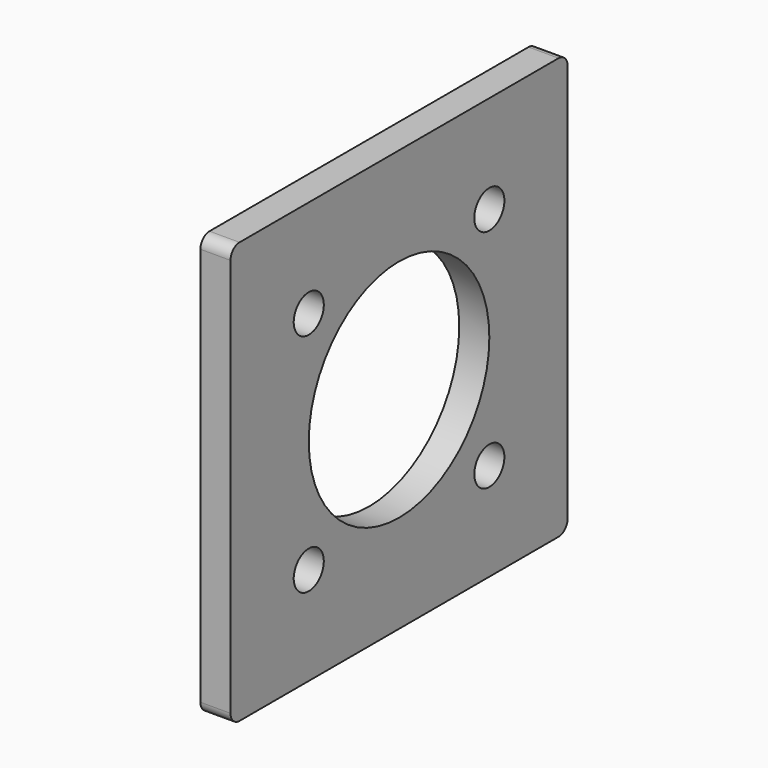
from build123d import *

# Parameters (mm, degrees)
F0_W     = 56
F0_H     = 56
F0_R     = 2.5
F0_R_2   = 15
F1_DEPTH = 4
F2_R     = 1.5


# Not quite as in the source:
# - a feature names something its author has since deleted; it is built from what else it names


with BuildPart() as f1:
    # F0 (on Right) → F1 (new body)
    with BuildSketch(Plane.YZ):
        Rectangle(F0_W, F0_H)
        with Locations((-15, -15)):
            Circle(F0_R, mode=Mode.SUBTRACT)
        with Locations((15, -15)):
            Circle(F0_R, mode=Mode.SUBTRACT)
        with Locations((-15, 15)):
            Circle(F0_R, mode=Mode.SUBTRACT)
        Circle(F0_R_2, mode=Mode.SUBTRACT)
        with Locations((15, 15)):
            Circle(F0_R, mode=Mode.SUBTRACT)
    extrude(amount=F1_DEPTH)

    # F2
    f2_edges = [f1.edges().sort_by_distance(p)[0] for p in [
        (2, -28, 28),
        (2, -28, -28),
        (2, 28, -28),
        (2, 28, 28),
    ]]
    fillet(f2_edges, radius=F2_R)


with BuildPart() as f3_1:
    # F3: copy of F1
    add(f1.part)


solid = f1.part
